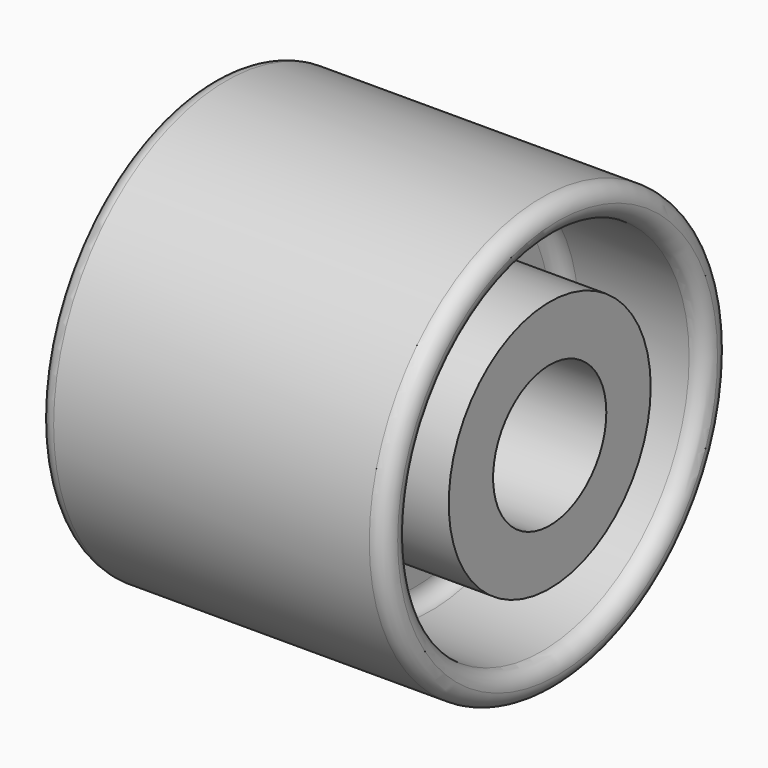
from build123d import *

# Parameters (mm, degrees)
F0_R     = 41
F0_R_2   = 35
F1_DEPTH = 33
F0_R_3   = 24
F0_R_4   = 13.45
F2_DEPTH = 31.5
F3_DEPTH = 6
F4_R     = 2.99999


# Not quite as in the source:
# - a fillet or chamfer is up to 0.001 mm smaller than in the source, because OpenCascade refuses the exact size


with BuildPart() as f1:
    # F0 (on Right) → F1 (new body, symmetric)
    with BuildSketch(Plane.YZ):
        Circle(F0_R)
        Circle(F0_R_2, mode=Mode.SUBTRACT)
    extrude(amount=F1_DEPTH, both=True)



with BuildPart() as f2:
    # F0 (on Right) → F2 (new body, symmetric)
    with BuildSketch(Plane.YZ):
        Circle(F0_R_3)
        Circle(F0_R_4, mode=Mode.SUBTRACT)
    extrude(amount=F2_DEPTH, both=True)


with BuildPart() as f1_1:
    add(f1.part)

    add(f2.part)  # F3 merges F2
    # F0 (on Right) → F3 (join, symmetric)
    with BuildSketch(Plane.YZ):
        Circle(F0_R_2)
        Circle(F0_R_3, mode=Mode.SUBTRACT)
    extrude(amount=F3_DEPTH, both=True)

    # F4 (radius 3 in the source; OpenCascade refuses exactly that, so slightly less here)
    f4_edges = [f1_1.edges().sort_by_distance(p)[0] for p in [
        (33, -35, 0),
        (6, -24, 0),
        (6, -35, 0),
        (33, -41, 0),
        (-6, -35, 0),
        (-6, -24, 0),
        (-33, -35, 0),
        (-33, -41, 0),
    ]]
    fillet(f4_edges, radius=F4_R)


solid = f1_1.part
